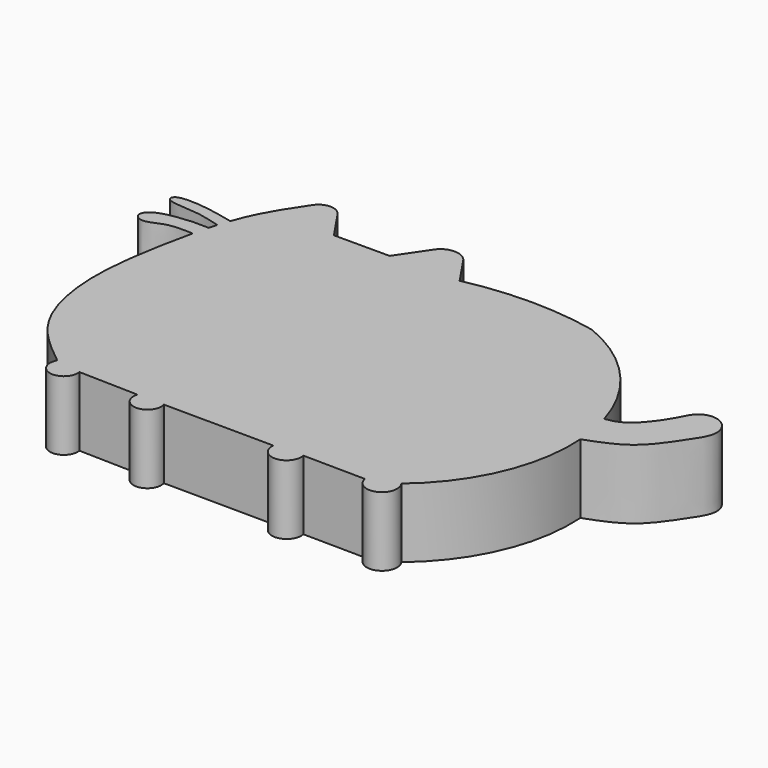
from build123d import *

# Parameters (mm, degrees)
F1_DEPTH = 5


with BuildPart() as f1:
    # F0 (on Top) → F1 (new body)
    with BuildSketch(Plane.XY):
        with BuildLine():
            add(Edge.make_bspline(
                [(-21.8114407323, -1.2526222444), (-21.9529955358, -1.8558107382), (-22.5042300878, -4.4975959061), (-23.2202782456, -9.1739987206), (-22.139771433, -14.0575578844), (-20.1089547521, -16.5186726713), (-18.7428019831, -17.6076660665), (-18.0927556227, -18.1258433528)],
                knots=[0.2898740891, 0.2898740891, 0.2898740891, 0.2898740891, 0.3516059803, 0.5530922378, 0.7304752816, 0.8716699309, 1, 1, 1, 1], degree=3))
            ThreePointArc((-18.0927556227, -18.1258433528), (-17.3935839447, -19.6099932849), (-16.2286459528, -18.4548043257))
            Line((-16.2286459528, -18.4548043257), (-11.9521580111, -18.5644586109))
            ThreePointArc((-11.9521580111, -18.5644586109), (-11.0039228875, -19.8642260207), (-10.0330017809, -18.5813162912))
            Line((-10.0330017809, -18.5813162912), (-2.0894149434, -18.6357257221))
            ThreePointArc((-2.0894149434, -18.6357257221), (-0.9857511229, -19.81017747), (0, -18.5351459173))
            Line((0, -18.5351459173), (4.4892215974, -18.5898928889))
            ThreePointArc((4.4892215974, -18.5898928889), (5.9989401794, -19.4034770666), (6.4432226901, -17.7470403905))
            ThreePointArc((6.4432226901, -17.7470403905), (9.9584459704, -13.0258381827), (10.9487174865, -7.2236052228))
            add(Edge.make_bspline(
                [(10.4463008096, -4.4422445204), (10.8741972144, -4.3675474393), (11.8690913168, -4.1773115011), (13.5331652433, -2.0119802219), (14.0806952433, -0.4605773182), (15.7511056613, -0.2652793882), (16.8446379611, -1.8141733756), (15.5062311575, -3.7223544079), (13.9418083475, -6.1089896659), (11.9710015695, -6.8499874791), (10.9487174865, -7.2236052228)],
                knots=[0, 0, 0, 0, 0.1032905111, 0.2470068386, 0.3581027377, 0.4596162524, 0.5663566268, 0.6946800325, 0.8436383674, 1, 1, 1, 1], degree=3))
            ThreePointArc((10.4463008096, -4.4422445204), (7.6865725324, 0.4345842042), (3.0868465244, 3.6349090665))
            ThreePointArc((3.0868465244, 3.6349090665), (-1.6830821707, 4.1394944322), (-6.4530108658, 3.6349090665))
            Line((-6.4530108658, 3.6349090665), (-7.8392599399, 5.6913481227))
            ThreePointArc((-7.8392599399, 5.6913481227), (-8.9107684121, 6.2612714829), (-9.9822768844, 5.6913481227))
            Line((-9.9822768844, 5.6913481227), (-11.4308783984, 3.5424119856))
            Line((-11.4308783984, 3.5424119856), (-15.4505299922, 3.5424119856))
            Line((-15.4505299922, 3.5424119856), (-16.9131534756, 5.6913481227))
            ThreePointArc((-16.9131534756, 5.6913481227), (-17.8046582966, 6.1629747599), (-18.6961631175, 5.6913481227))
            add(Edge.make_bspline(
                [(-18.6961631175, 5.6913481227), (-19.4285369113, 4.6153397899), (-20.3296673033, 3.2727021769), (-20.9824057089, 1.5831681063), (-21.0991354999, 1.2502842354)],
                knots=[0, 0, 0, 0, 0.1619455579, 0.2001015887, 0.2001015887, 0.2001015887, 0.2001015887], degree=3))
            add(Edge.make_bspline(
                [(-21.0991354999, 1.2502842354), (-21.1939808519, 0.9798092551), (-21.2837186334, 0.7022584), (-21.3690435276, 0.4186483175)],
                knots=[0.2001015887, 0.2001015887, 0.2001015887, 0.2001015887, 0.2311041471, 0.2311041471, 0.2311041471, 0.2311041471], degree=3))
            add(Edge.make_bspline(
                [(-21.3690435276, 0.4186483175), (-21.4258706707, 0.2297614645), (-21.4807403986, 0.0381869326), (-21.5338579347, -0.15577494)],
                knots=[0.2311041471, 0.2311041471, 0.2311041471, 0.2311041471, 0.2517521285, 0.2517521285, 0.2517521285, 0.2517521285], degree=3))
            add(Edge.make_bspline(
                [(-21.5338579347, -0.15577494), (-21.6319277937, -0.5138829189), (-21.7240248677, -0.8801287474), (-21.8114407323, -1.2526222444)],
                knots=[0.2517521285, 0.2517521285, 0.2517521285, 0.2517521285, 0.2898740891, 0.2898740891, 0.2898740891, 0.2898740891], degree=3))
        make_face()
        with BuildLine():
            add(Edge.make_bspline(
                [(-21.5338579347, -0.15577494), (-22.2120015737, -0.1084108073), (-23.5399972583, -0.1535762915), (-25.3752977452, -0.5600385686), (-25.8170028342, -1.4584373864), (-24.9213051104, -1.9865694968), (-23.7099288456, -1.1824261792), (-22.4818931077, -1.2268881647), (-21.8114407323, -1.2526222444)],
                knots=[0, 0, 0, 0, 0.2053222205, 0.3970043755, 0.5164824715, 0.6375428035, 0.802694074, 1, 1, 1, 1], degree=3))
            add(Edge.make_bspline(
                [(-21.5338579347, -0.15577494), (-21.6319277937, -0.5138829189), (-21.7240248677, -0.8801287474), (-21.8114407323, -1.2526222444)],
                knots=[0.2517521285, 0.2517521285, 0.2517521285, 0.2517521285, 0.2898740891, 0.2898740891, 0.2898740891, 0.2898740891], degree=3))
        make_face()
        with BuildLine():
            add(Edge.make_bspline(
                [(-21.0991354999, 1.2502842354), (-21.9336416547, 1.4389735678), (-23.4277348773, 1.7756429479), (-25.1450687292, 1.7862361389), (-25.5103505424, 1.4724239125), (-25.4694238607, 1.0699461681), (-24.2868908085, 0.8974097249), (-22.8783994531, 0.8784133331), (-21.8863935379, 0.5464820129), (-21.3690435276, 0.4186483175)],
                knots=[0, 0, 0, 0, 0.2119793639, 0.3816308644, 0.4632349714, 0.5312430576, 0.6687854633, 0.8325027876, 1, 1, 1, 1], degree=3))
            add(Edge.make_bspline(
                [(-21.0991354999, 1.2502842354), (-21.1939808519, 0.9798092551), (-21.2837186334, 0.7022584), (-21.3690435276, 0.4186483175)],
                knots=[0.2001015887, 0.2001015887, 0.2001015887, 0.2001015887, 0.2311041471, 0.2311041471, 0.2311041471, 0.2311041471], degree=3))
        make_face()
    extrude(amount=F1_DEPTH)


solid = f1.part
